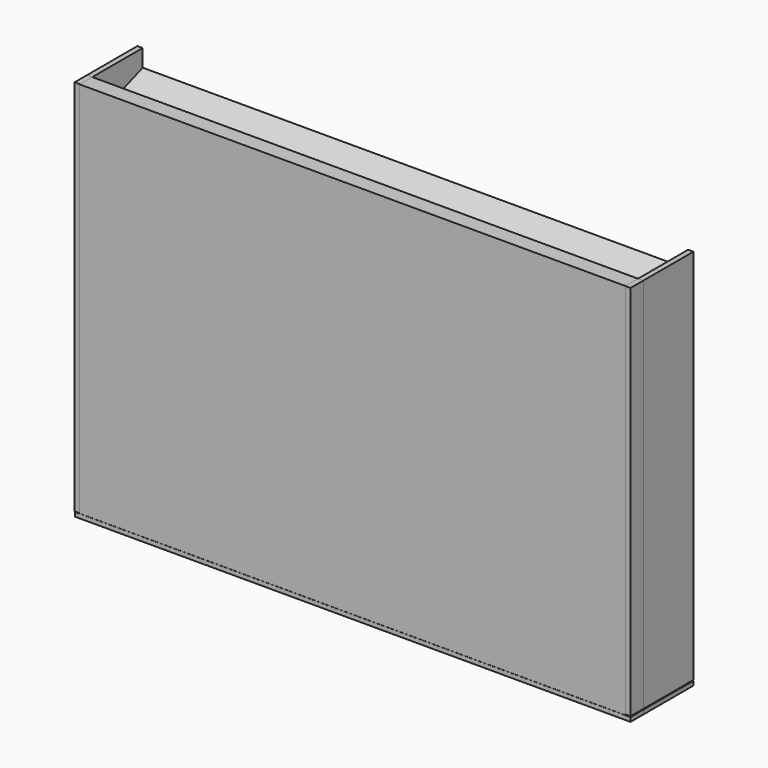
from build123d import *

# Parameters (mm, degrees)
F0_W      = 9.5758
F0_H      = 228.6
F1_DEPTH  = 330.2
F3_DEPTH  = 330.2
F4_W      = 38.0470480231
F4_H      = 228.509646448
F5_DEPTH  = 3.175
F6_W      = 37.8971553801
F6_H      = 228.1222460593
F7_DEPTH  = 3.175
F8_W      = 336.1774778459
F8_H      = 37.8997616915
F9_DEPTH  = 2.54
F10_DEPTH = 9.398
F11_DEPTH = 9.652
F12_DEPTH = 9.652


# Not quite as in the source:
# - a feature names something its author has since deleted; it is built from what else it names


with BuildPart() as f1:
    # F0 (on Right) → F1 (new body)
    with BuildSketch(Plane.YZ):
        with Locations((-20.647819831, 59.7378891851)):
            Rectangle(F0_W, F0_H)
    extrude(amount=-F1_DEPTH)

    # F2 (on Right) → F3 (join)
    with BuildSketch(Plane.YZ):
        Polygon((22.0372355491, -26.9659241096), (-16.0627644509, -40.8476963639), (-16.0627644509, -42.7134521306), (22.0372355491, -28.8960468024), align=None)
        Polygon((22.1871281922, 36.5340758904), (-15.9128718078, 20.7688752562), (-15.9128718078, 18.928617239), (22.1871281922, 34.6444733441), align=None)
        Polygon((22.1694405138, 100.0340758904), (-15.9305594862, 81.9853842258), (-15.9305594862, 80.1339223981), (22.1694405138, 98.1948003173), align=None)
    extrude(amount=-F3_DEPTH)


with BuildPart() as f3:
    # F2 (on Right) → F3, piece 2 (new body)
    with BuildSketch(Plane.YZ):
        Polygon((22.2718652983, 163.5340758904), (-15.8281347017, 149.7193872929), (-15.8281347017, 147.5223718815), (22.2718652983, 161.3244234257), align=None)
    extrude(amount=-F3_DEPTH)


with BuildPart() as f5:
    # F4 (on face) → F5 (new body)
    with BuildSketch(Plane(origin=(-330.2, 0, 0), x_dir=(0, -1, 0), z_dir=(-1, 0, 0))):
        with Locations((-3.1636041806, 59.7830659611)):
            Rectangle(F4_W, F4_H)
    extrude(amount=F5_DEPTH)


with BuildPart() as f7:
    # F6 (on face) → F7 (new body)
    with BuildSketch(Plane.YZ):
        with Locations((3.0886578591, 59.9767661554)):
            Rectangle(F6_W, F6_H)
    extrude(amount=F7_DEPTH)


with BuildPart() as f9:
    # F8 (on face) → F9 (new body)
    with BuildSketch(Plane(origin=(0, 0, -54.5621108149), x_dir=(1, 0, 0), z_dir=(0, 0, -1))):
        with Locations((-164.9049472762, -3.0899610148)):
            Rectangle(F8_W, F8_H)
    extrude(amount=F9_DEPTH)


with BuildPart() as f10:
    # F10 (new): a face of the model
    f10_faces = [f5.part.faces().sort_by_distance(p)[0] for p in [
        (-331.7875, -15.859919831, 59.7830659611),
    ]]
    extrude(f10_faces, amount=F10_DEPTH)


with BuildPart() as f11:
    # F11 (new): a face of the model
    f11_faces = [f9.part.faces().sort_by_distance(p)[0] for p in [
        (-164.9049472762, -15.859919831, -55.8321108149),
    ]]
    extrude(f11_faces, amount=F11_DEPTH)


with BuildPart() as f12:
    # F12 (new): a face of the model
    f12_faces = [f7.part.faces().sort_by_distance(p)[0] for p in [
        (1.5875, -15.859919831, 59.9767661554),
    ]]
    extrude(f12_faces, amount=F12_DEPTH)


solid = Compound([f1.part, f3.part, f5.part, f7.part, f9.part, f10.part, f11.part, f12.part])
